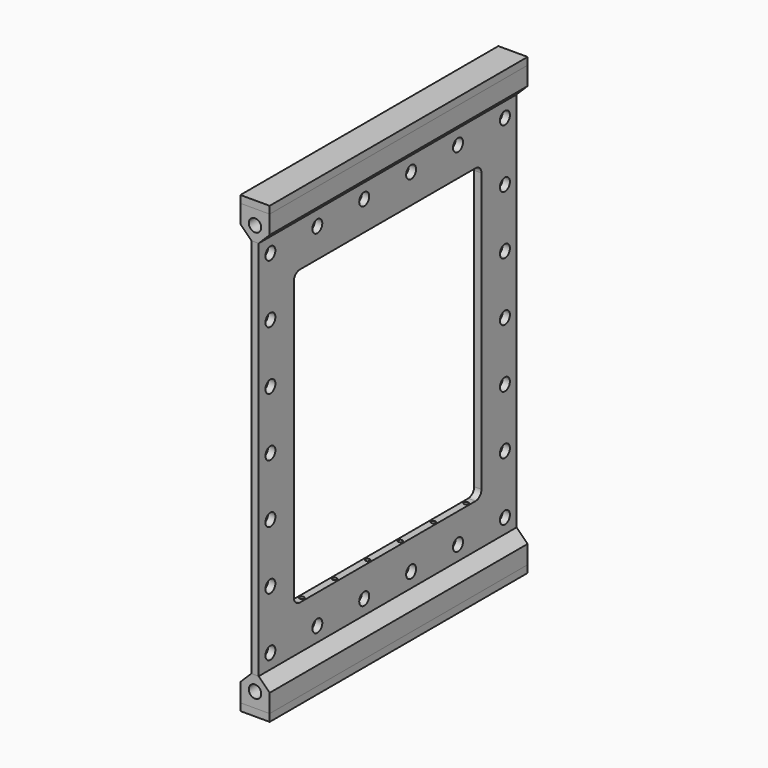
from build123d import *

# Parameters (mm, degrees)
F0_W        = 220
F0_H        = 260
F0_R        = 4.25
F0_W_2      = 160
F0_H_2      = 200
F1_DEPTH    = 2.5
F2_W        = 20
F2_H        = 20
F3_DEPTH    = 220
F4_W        = 10
F4_H        = 180
F5_DEPTH    = 15
F6_R        = 4.99999
F7_SIZE     = 7.5
F9_D        = 8.5
F9_DEPTH    = 29.5
F9_TIP      = 2.5536576309
F4_W_2      = 20
F4_H_2      = 220
F11_DEPTH   = 5
F13_D       = 3
F13_DEPTH   = 35
F13_TIP     = 0.9012909285
F13_2_D     = 3
F13_2_DEPTH = 35
F13_2_TIP   = 0.9012909285
F15_D       = 3
F15_DEPTH   = 35
F15_TIP     = 0.9012909285
F15_2_D     = 3
F15_2_DEPTH = 35
F15_2_TIP   = 0.9012909285
F17_R       = 5


# Not quite as in the source:
# - a fillet or chamfer is up to 0.001 mm smaller than in the source, because OpenCascade refuses the exact size


with BuildPart() as f1:
    # F0 (on Right) → F1 (new body, symmetric)
    with BuildSketch(Plane.YZ):
        Rectangle(F0_W, F0_H)
        with Locations((-100, -120)):
            Circle(F0_R, mode=Mode.SUBTRACT)
        with Locations((-60, -120)):
            Circle(F0_R, mode=Mode.SUBTRACT)
        with Locations((-100, -80)):
            Circle(F0_R, mode=Mode.SUBTRACT)
        with Locations((-20, -120)):
            Circle(F0_R, mode=Mode.SUBTRACT)
        with Locations((-100, -40)):
            Circle(F0_R, mode=Mode.SUBTRACT)
        with Locations((20, -120)):
            Circle(F0_R, mode=Mode.SUBTRACT)
        with Locations((60, -120)):
            Circle(F0_R, mode=Mode.SUBTRACT)
        with Locations((100, -120)):
            Circle(F0_R, mode=Mode.SUBTRACT)
        with Locations((100, -80)):
            Circle(F0_R, mode=Mode.SUBTRACT)
        with Locations((100, -40)):
            Circle(F0_R, mode=Mode.SUBTRACT)
        with Locations((-100, 0)):
            Circle(F0_R, mode=Mode.SUBTRACT)
        with Locations((-100, 40)):
            Circle(F0_R, mode=Mode.SUBTRACT)
        with Locations((-100, 80)):
            Circle(F0_R, mode=Mode.SUBTRACT)
        with Locations((-100, 120)):
            Circle(F0_R, mode=Mode.SUBTRACT)
        with Locations((-60, 120)):
            Circle(F0_R, mode=Mode.SUBTRACT)
        with Locations((-20, 120)):
            Circle(F0_R, mode=Mode.SUBTRACT)
        Rectangle(F0_W_2, F0_H_2, mode=Mode.SUBTRACT)
        with Locations((100, 0)):
            Circle(F0_R, mode=Mode.SUBTRACT)
        with Locations((100, 40)):
            Circle(F0_R, mode=Mode.SUBTRACT)
        with Locations((20, 120)):
            Circle(F0_R, mode=Mode.SUBTRACT)
        with Locations((100, 80)):
            Circle(F0_R, mode=Mode.SUBTRACT)
        with Locations((60, 120)):
            Circle(F0_R, mode=Mode.SUBTRACT)
        with Locations((100, 120)):
            Circle(F0_R, mode=Mode.SUBTRACT)
    extrude(amount=F1_DEPTH, both=True)

    # F13 (one way)
    with BuildSketch(Plane(origin=(0, 0, 100), x_dir=(1, 0, 0), z_dir=(0, 0, -1))):
        with Locations((0, -70), (0, -42), (0, -14), (0, 14), (0, 42), (0, 70)):
            Circle(F13_D / 2)
    extrude(amount=-F13_DEPTH, mode=Mode.SUBTRACT)
    with Locations(Plane(origin=(0, 0, 100), x_dir=(1, 0, 0), z_dir=(0, 0, -1))):
        with Locations((0, -70), (0, -42), (0, -14), (0, 14), (0, 42), (0, 70)):
            with Locations((0, 0, -(F13_DEPTH + F13_TIP / 2))):  # 118° drill point
                Cone(0, F13_D / 2, F13_TIP, mode=Mode.SUBTRACT)

    # F15
    with Locations(Plane.XY.offset(-100)):
        with Locations((0, 70), (0, 42), (0, 14), (0, -14), (0, -42), (0, -70)):
            Hole(F15_D / 2, depth=F15_DEPTH)
            with Locations((0, 0, -(F15_DEPTH + F15_TIP / 2))):  # 118° drill point
                Cone(0, F15_D / 2, F15_TIP, mode=Mode.SUBTRACT)

    # F17
    f17_edges = [f1.edges().sort_by_distance(p)[0] for p in [
        (0, 80, 100),
        (0, -80, 100),
        (0, 80, -100),
        (0, -80, -100),
    ]]
    fillet(f17_edges, radius=F17_R)


with BuildPart() as f3:
    # F2 (on face) → F3 (new body)
    with BuildSketch(Plane.XZ.offset(110)):
        with Locations((0, 140)):
            Rectangle(F2_W, F2_H)
    extrude(amount=-F3_DEPTH)

    # F4 (on face) → F5 (cut)
    with BuildSketch(Plane.XY.offset(150)):
        Rectangle(F4_W, F4_H)
    extrude(amount=-F5_DEPTH, mode=Mode.SUBTRACT)

    # F6 (radius 5 in the source; OpenCascade refuses exactly that, so slightly less here)
    f6_edges = [f3.edges().sort_by_distance(p)[0] for p in [
        (-5, 0, 135),
        (0, -90, 135),
        (5, 0, 135),
        (0, 90, 135),
        (-5, 90, 142.5),
        (5, 90, 142.5),
        (-5, -90, 142.5),
        (5, -90, 142.5),
    ]]
    fillet(f6_edges, radius=F6_R)

    # F7
    f7_edges = [f3.edges().sort_by_distance(p)[0] for p in [
        (10, 0, 130),
        (-10, 0, 130),
    ]]
    chamfer(f7_edges, length=F7_SIZE)

    # F9
    with Locations(Plane.XZ.offset(110)):
        with Locations((0, 140)):
            Hole(F9_D / 2, depth=F9_DEPTH)
            with Locations((0, 0, -(F9_DEPTH + F9_TIP / 2))):  # 118° drill point
                Cone(0, F9_D / 2, F9_TIP, mode=Mode.SUBTRACT)


with BuildPart() as f10_1:
    # F10: instance of F3
    add(f3.part.mirror(Plane.XY))

    # F15#2
    with Locations(Plane.XY.offset(-100)):
        with Locations((0, 70), (0, 42), (0, 14), (0, -14), (0, -42), (0, -70)):
            Hole(F15_2_D / 2, depth=F15_2_DEPTH)
            with Locations((0, 0, -(F15_2_DEPTH + F15_2_TIP / 2))):  # 118° drill point
                Cone(0, F15_2_D / 2, F15_2_TIP, mode=Mode.SUBTRACT)


with BuildPart() as f11:
    # F4 (on face) → F11 (new body)
    with BuildSketch(Plane.XY.offset(150)):
        Rectangle(F4_W_2, F4_H_2)
        Rectangle(F4_W, F4_H, mode=Mode.SUBTRACT)
        Rectangle(F4_W, F4_H)
    extrude(amount=F11_DEPTH)


with BuildPart() as f3_1:
    add(f3.part)

    # F13#2 (one way)
    with BuildSketch(Plane(origin=(0, 0, 100), x_dir=(1, 0, 0), z_dir=(0, 0, -1))):
        with Locations((0, -70), (0, -42), (0, -14), (0, 14), (0, 42), (0, 70)):
            Circle(F13_2_D / 2)
    extrude(amount=-F13_2_DEPTH, mode=Mode.SUBTRACT)
    with Locations(Plane(origin=(0, 0, 100), x_dir=(1, 0, 0), z_dir=(0, 0, -1))):
        with Locations((0, -70), (0, -42), (0, -14), (0, 14), (0, 42), (0, 70)):
            with Locations((0, 0, -(F13_2_DEPTH + F13_2_TIP / 2))):  # 118° drill point
                Cone(0, F13_2_D / 2, F13_2_TIP, mode=Mode.SUBTRACT)


with BuildPart() as f16_1:
    # F16: instance of F11
    add(f11.part.mirror(Plane.XY))


solid = Compound([f1.part, f10_1.part, f11.part, f3_1.part, f16_1.part])
